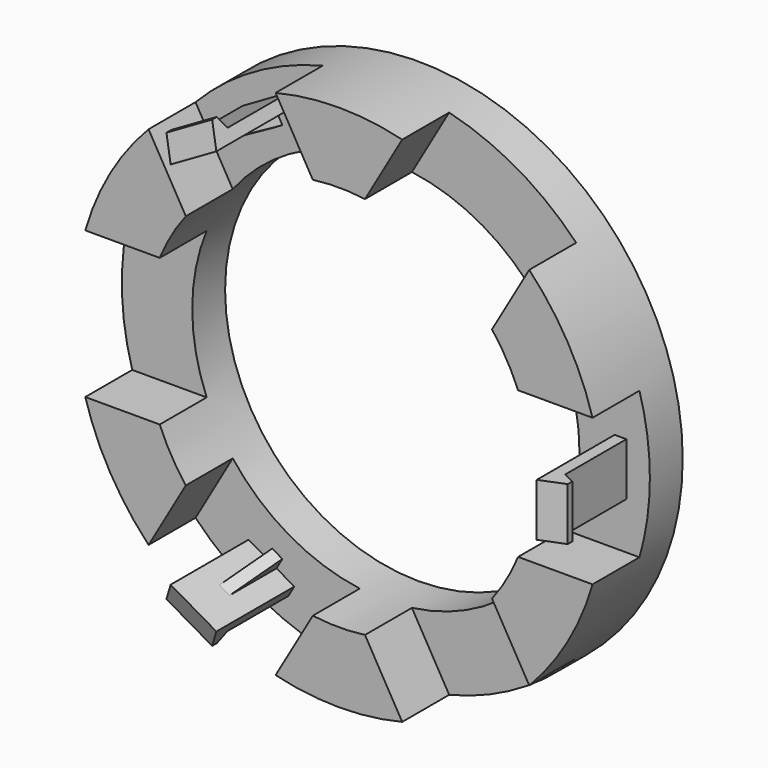
from build123d import *

# Parameters (mm, degrees)
F0_R             = 45
F0_R_2           = 33
F1_DEPTH         = 17
F2_R             = 5
F3_DEPTH         = 0.5
F3_COPIES_COUNT  = 6
F6_DEPTH         = 10
F8_COUNT         = 6
F9_W             = 6
F9_H             = 9
F10_DEPTH        = 17
F10_COPIES_COUNT = 3
F12_DEPTH        = 10
F12_COPIES_COUNT = 3
F14_DEPTH        = 1
F14_COPIES_COUNT = 3


# Not quite as in the source:
# - a pattern or mirror of a feature is missing from the dataset's text; its kind, count and spacing are read off the source's solid
# - a feature names something its author has since deleted; it is built from what else it names


with BuildPart() as f1:
    # F0 (on Front) → F1 (new body)
    with BuildSketch(Plane.XZ):
        Circle(F0_R)
        Circle(F0_R_2, mode=Mode.SUBTRACT)
    extrude(amount=F1_DEPTH)

    # F2 (on Front) → F3 (cut)
    with BuildSketch(Plane.XZ):
        with Locations((0, 39)):
            Circle(F2_R)
    f3 = extrude(amount=F3_DEPTH, mode=Mode.SUBTRACT)

    # F3_copies: F3 ×6 about axis
    f3_copies_axis = Axis((0, 0, 0), (0, 1, 0))
    for i in range(1, F3_COPIES_COUNT):
        add(f3.rotate(f3_copies_axis, i * 360 / F3_COPIES_COUNT), mode=Mode.SUBTRACT)

    # F5 (on face) → F6 (cut)
    with BuildSketch(Plane.XZ.offset(17)):
        with BuildLine():
            Line((-30.5409561082, 12.5), (-43.2290411645, 12.5))
            ThreePointArc((-43.2290411645, 12.5), (-45, 0), (-43.2290411645, -12.5))
            Line((-43.2290411645, -12.5), (-30.5409561082, -12.5))
            ThreePointArc((-30.5409561082, -12.5), (-33, 0), (-30.5409561082, 12.5))
        make_face()
    f6 = extrude(amount=-F6_DEPTH, mode=Mode.SUBTRACT)

    # F8: F6 ×6 about axis
    f8_axis = Axis((0, -20.116, 0), (0, -1, 0))
    for i in range(1, F8_COUNT):
        add(f6.rotate(f8_axis, i * 360 / F8_COUNT), mode=Mode.SUBTRACT)

    # F9 (on face) → F10 (join)
    with BuildSketch(Plane.XZ.offset(7)):
        with Locations((42, 0)):
            Rectangle(F9_W, F9_H)
    f10 = extrude(amount=F10_DEPTH)

    # F10_copies: F10 ×3 about axis
    f10_copies_axis = Axis((0, 0, 0), (0, 1, 0))
    for i in range(1, F10_COPIES_COUNT):
        add(f10.rotate(f10_copies_axis, i * 360 / F10_COPIES_COUNT))

    # F11 (on face) → F12 (cut)
    with BuildSketch(Plane(origin=(0, 0, -4.5), x_dir=(1, 0, 0), z_dir=(0, 0, -1))):
        Polygon((39, 24), (39, 23.6), (43, 22), (43, 21), (41, 20), (41, 7), (44.7744346698, 7), (45, 7), (45, 24), align=None)
    f12 = extrude(amount=-F12_DEPTH, mode=Mode.SUBTRACT)

    # F12_copies: F12 ×3 about axis
    f12_copies_axis = Axis((0, 0, 0), (0, 1, 0))
    for i in range(1, F12_COPIES_COUNT):
        add(f12.rotate(f12_copies_axis, i * 360 / F12_COPIES_COUNT), mode=Mode.SUBTRACT)

    # F13 (on Top) → F14 (join, symmetric)
    with BuildSketch(Plane.XY):
        Polygon((37, -7), (39, -17), (39, -7), align=None)
    f14 = extrude(amount=F14_DEPTH, both=True)

    # F14_copies: F14 ×3 about axis
    f14_copies_axis = Axis((0, 0, 0), (0, 1, 0))
    for i in range(1, F14_COPIES_COUNT):
        add(f14.rotate(f14_copies_axis, i * 360 / F14_COPIES_COUNT))


solid = f1.part
